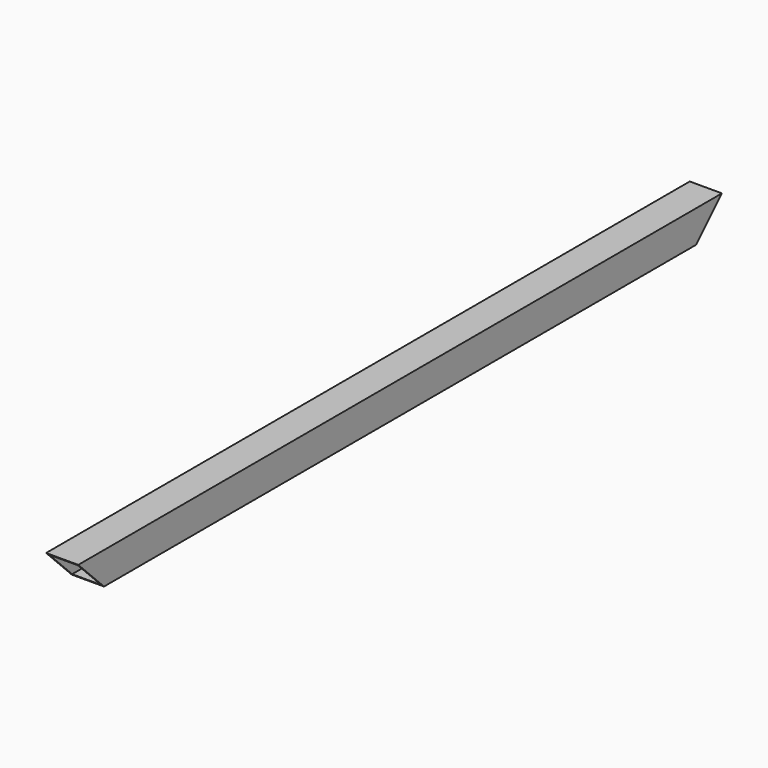
from build123d import *

# Parameters (mm, degrees)
F0_W        = 40
F0_H        = 40
F1_DEPTH    = 1000
F2_W        = 36
F2_H        = 36
F3_DEPTH    = 1000.001
F4_T1_DEPTH = 245.7346390373


# Not quite as in the source:
# - a fillet or chamfer that OpenCascade refuses, or shapes differently, is made with other operations: its cross-section is extruded or revolved along the edge and cut away or added


with BuildPart() as f1:
    # F0 (on Front) → F1 (new body)
    with BuildSketch(Plane.XZ):
        with Locations((20, 20)):
            Rectangle(F0_W, F0_H)
    extrude(amount=F1_DEPTH)

    # F2 (on face) → F3 (cut, through all)
    with BuildSketch(Plane.XZ.offset(1000)):
        with Locations((20, 20)):
            Rectangle(F2_W, F2_H)
    extrude(amount=-F3_DEPTH, mode=Mode.SUBTRACT)

    # F4: chamfer of 40 on 2 edges, made by hand

    # F4_s2 → F4_t1 (cut)
    with BuildSketch(Plane.YZ.offset(-102.8673195186)):
        Polygon((-960, 0), (-1000, 40), (-1000, 0), align=None)
        Polygon((-40, 0), (0, 40), (0, 0), align=None)
    extrude(amount=F4_T1_DEPTH, mode=Mode.SUBTRACT)


solid = f1.part
